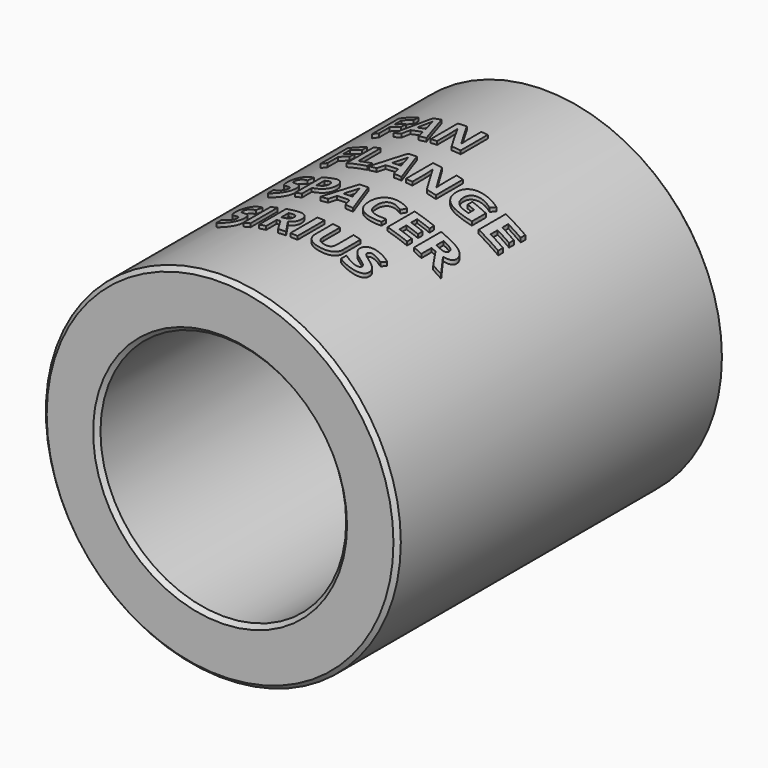
from build123d import *

# Parameters (mm, degrees)
F0_R         = 26
F0_R_2       = 18
F1_DEPTH     = 60
F2_SIZE      = 0.6
F4_TEXT_SIZE = 6.9444444444
F6_R         = 35
F6_R_2       = 26.5
F7_DEPTH     = 60.001


# Not quite as in the source:
# - Text() gives the source's letters only with a copy of the font that has no kerning and outlines rounded to 1/6400 em; it was checked with that copy


with BuildPart() as f1:
    # F0 (on Front) → F1 (new body)
    with BuildSketch(Plane.XZ):
        Circle(F0_R)
        Circle(F0_R_2, mode=Mode.SUBTRACT)
    extrude(amount=F1_DEPTH)

    # F2
    f2_edges = [f1.edges().sort_by_distance(p)[0] for p in [
        (-26, 0, 0),
        (-18, 0, 0),
        (-18, -60, 0),
        (-26, -60, 0),
    ]]
    chamfer(f2_edges, length=F2_SIZE)

    # F4 (on offset) → F5 (join, up to the next surface of F1)
    with BuildSketch(Plane.XY.offset(30)):
        with Locations((-11.253143491, -18.9001597772)):
            Text('FAN', F4_TEXT_SIZE, font='Open Sans', font_style=FontStyle.BOLD, text_align=(TextAlign.LEFT, TextAlign.BOTTOM))
        with Locations((-11.253143491, -28.3446042217)):
            Text('FLANGE', F4_TEXT_SIZE, font='Open Sans', font_style=FontStyle.BOLD, text_align=(TextAlign.LEFT, TextAlign.BOTTOM))
        with Locations((-11.253143491, -37.7890486661)):
            Text('SPACER', F4_TEXT_SIZE, font='Open Sans', font_style=FontStyle.BOLD, text_align=(TextAlign.LEFT, TextAlign.BOTTOM))
        with Locations((-11.253143491, -47.2334931106)):
            Text('SIRIUS', F4_TEXT_SIZE, font='Open Sans', font_style=FontStyle.BOLD, text_align=(TextAlign.LEFT, TextAlign.BOTTOM))
    extrude(until=Until.NEXT, dir=(0, 0, -1))

    # F6 (on face) → F7 (cut, through all)
    with BuildSketch(Plane(origin=(0, 0, 0), x_dir=(-1, 0, 0), z_dir=(0, 1, 0))):
        Circle(F6_R)
        Circle(F6_R_2, mode=Mode.SUBTRACT)
    extrude(amount=-F7_DEPTH, mode=Mode.SUBTRACT)


solid = f1.part
